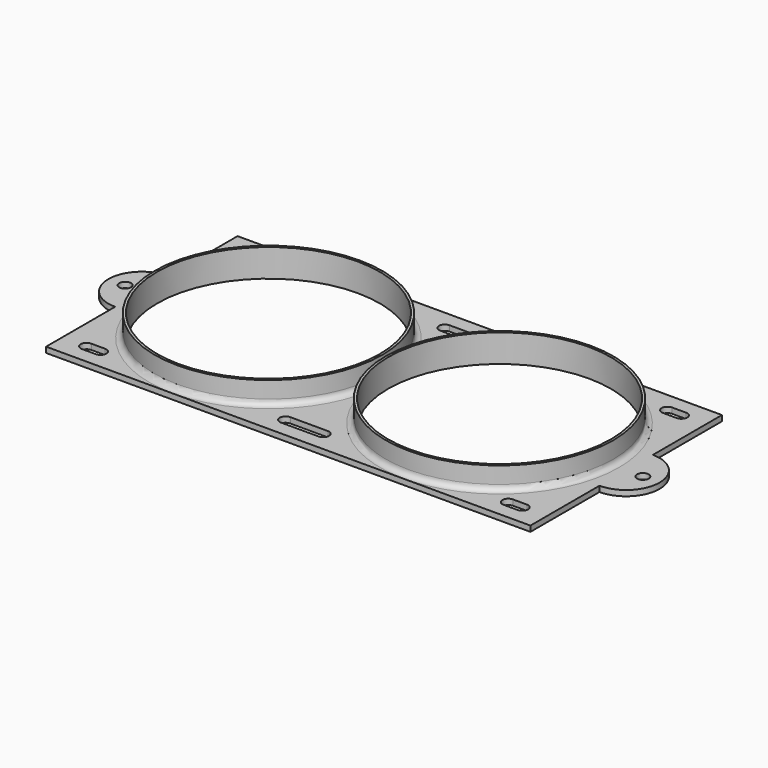
from build123d import *

# Parameters (mm, degrees)
F0_R     = 40.88
F0_R_2   = 2.1
F0_R_3   = 40
F1_DEPTH = 2
F2_DEPTH = 10


# Not quite as in the source:
# - a fillet or chamfer that OpenCascade refuses, or shapes differently, is made with other operations: its cross-section is extruded or revolved along the edge and cut away or added


with BuildPart() as f1:
    # F0 (on Top) → F1 (new body)
    with BuildSketch(Plane.XY):
        with BuildLine():
            Line((-41.5, -43), (41.5, -43))
            Line((41.5, -43), (41.5, 43))
            Line((41.5, 43), (-41.5, 43))
            Line((-41.5, 43), (-41.5, 37.85))
            Line((-41.5, 37.85), (-34.75, 37.85))
            ThreePointArc((-34.75, 37.85), (-32.65, 35.75), (-34.75, 33.65))
            Line((-34.75, 33.65), (-41.5, 33.65))
            Line((-41.5, 33.65), (-41.5, -33.65))
            Line((-41.5, -33.65), (-34.75, -33.65))
            ThreePointArc((-34.75, -33.65), (-32.65, -35.75), (-34.75, -37.85))
            Line((-34.75, -37.85), (-41.5, -37.85))
            Line((-41.5, -37.85), (-41.5, -43))
        make_face()
        with BuildLine():
            ThreePointArc((36.75, -33.65), (38.85, -35.75), (36.75, -37.85))
            Line((36.75, -37.85), (31.75, -37.85))
            ThreePointArc((31.75, -37.85), (29.65, -35.75), (31.75, -33.65))
            Line((31.75, -33.65), (36.75, -33.65))
        make_face(mode=Mode.SUBTRACT)
        Circle(F0_R, mode=Mode.SUBTRACT)
        with BuildLine():
            Line((31.75, 37.85), (36.75, 37.85))
            ThreePointArc((36.75, 37.85), (38.85, 35.75), (36.75, 33.65))
            Line((36.75, 33.65), (31.75, 33.65))
            ThreePointArc((31.75, 33.65), (29.65, 35.75), (31.75, 37.85))
        make_face(mode=Mode.SUBTRACT)
        Polygon((41.5, 43), (41.5, -43), (45.5, -43), (45.5, -12), (45.5, 12), (45.5, 43), align=None)
        with BuildLine():
            Line((-124.5, -43), (-41.5, -43))
            Line((-41.5, -43), (-41.5, -37.85))
            Line((-41.5, -37.85), (-48.25, -37.85))
            ThreePointArc((-48.25, -37.85), (-50.35, -35.75), (-48.25, -33.65))
            Line((-48.25, -33.65), (-41.5, -33.65))
            Line((-41.5, -33.65), (-41.5, 33.65))
            Line((-41.5, 33.65), (-48.25, 33.65))
            ThreePointArc((-48.25, 33.65), (-50.35, 35.75), (-48.25, 37.85))
            Line((-48.25, 37.85), (-41.5, 37.85))
            Line((-41.5, 37.85), (-41.5, 43))
            Line((-41.5, 43), (-124.5, 43))
            Line((-124.5, 43), (-124.5, -43))
        make_face()
        with BuildLine():
            Line((-114.75, -37.85), (-119.75, -37.85))
            ThreePointArc((-119.75, -37.85), (-121.85, -35.75), (-119.75, -33.65))
            Line((-119.75, -33.65), (-114.75, -33.65))
            ThreePointArc((-114.75, -33.65), (-112.65, -35.75), (-114.75, -37.85))
        make_face(mode=Mode.SUBTRACT)
        with Locations((-83, 0)):
            Circle(F0_R, mode=Mode.SUBTRACT)
        with BuildLine():
            ThreePointArc((-119.75, 33.65), (-121.85, 35.75), (-119.75, 37.85))
            Line((-119.75, 37.85), (-114.75, 37.85))
            ThreePointArc((-114.75, 37.85), (-112.65, 35.75), (-114.75, 33.65))
            Line((-114.75, 33.65), (-119.75, 33.65))
        make_face(mode=Mode.SUBTRACT)
        Polygon((-128.5, -43), (-124.5, -43), (-124.5, 43), (-128.5, 43), (-128.5, 12), (-128.5, -12), align=None)
        with BuildLine():
            Line((45.5, 12), (45.5, -12))
            ThreePointArc((45.5, -12), (57.5, 0), (45.5, 12))
        make_face()
        with Locations((51.5, 0)):
            Circle(F0_R_2, mode=Mode.SUBTRACT)
        with BuildLine():
            ThreePointArc((-128.5, 12), (-140.5, 0), (-128.5, -12))
            Line((-128.5, -12), (-128.5, 12))
        make_face()
        with Locations((-134.5, 0)):
            Circle(F0_R_2, mode=Mode.SUBTRACT)
        Circle(F0_R)
        Circle(F0_R_3, mode=Mode.SUBTRACT)
        with Locations((-83, 0)):
            Circle(F0_R)
        with Locations((-83, 0)):
            Circle(F0_R_3, mode=Mode.SUBTRACT)
    extrude(amount=F1_DEPTH)

    # F0 (on Top) → F2 (join)
    with BuildSketch(Plane.XY):
        Circle(F0_R)
        Circle(F0_R_3, mode=Mode.SUBTRACT)
        with Locations((-83, 0)):
            Circle(F0_R)
        with Locations((-83, 0)):
            Circle(F0_R_3, mode=Mode.SUBTRACT)
    extrude(amount=F2_DEPTH)

    # F3: fillet of radius 2 on 2 edges, made by hand

    # F3_s1 → F3_t2 (revolve)
    with BuildSketch(Plane.XZ):
        with BuildLine():
            ThreePointArc((-40.12, 2), (-41.5342135624, 2.5857864376), (-42.12, 4))
            Line((-42.12, 4), (-42.12, 2))
            Line((-42.12, 2), (-40.12, 2))
        make_face()
    revolve(axis=Axis((-83, 0, 2), (0, 0, -1)))

    # F3_s3 → F3_t4 (revolve)
    with BuildSketch(Plane.XZ):
        with BuildLine():
            ThreePointArc((42.88, 2), (41.4657864376, 2.5857864376), (40.88, 4))
            Line((40.88, 4), (40.88, 2))
            Line((40.88, 2), (42.88, 2))
        make_face()
    revolve(axis=Axis((0, 0, 2), (0, 0, -1)))


solid = f1.part
